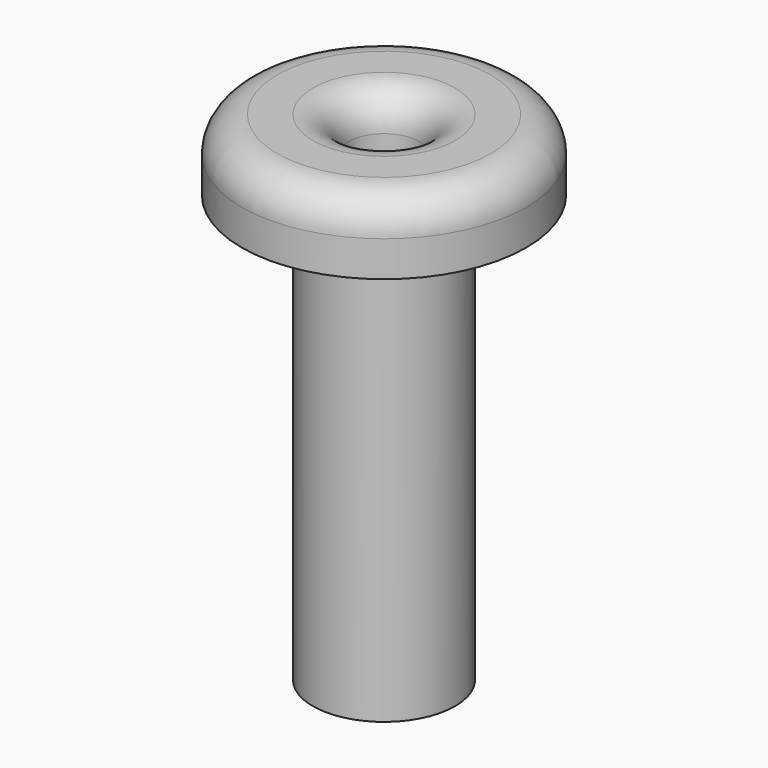
from build123d import *

# Parameters (mm, degrees)
F0_R     = 10
F0_R_2   = 2.5
F1_DEPTH = 5
F2_R     = 5
F2_R_2   = 2.5
F3_DEPTH = 30
F4_R     = 2.49999


# Not quite as in the source:
# - a fillet or chamfer is up to 0.001 mm smaller than in the source, because OpenCascade refuses the exact size


with BuildPart() as f1:
    # F0 (on Top) → F1 (new body)
    with BuildSketch(Plane.XY):
        Circle(F0_R)
        Circle(F0_R_2, mode=Mode.SUBTRACT)
    extrude(amount=F1_DEPTH)

    # F2 (on face) → F3 (join)
    with BuildSketch(Plane(origin=(0, 0, 0), x_dir=(1, 0, 0), z_dir=(0, 0, -1))):
        Circle(F2_R)
        Circle(F2_R_2, mode=Mode.SUBTRACT)
    extrude(amount=F3_DEPTH)

    # F4 (radius 2.5 in the source; OpenCascade refuses exactly that, so slightly less here)
    f4_edges = [f1.edges().sort_by_distance(p)[0] for p in [
        (-10, 0, 5),
        (-2.5, 0, 5),
        (-2.5, 0, -30),
    ]]
    fillet(f4_edges, radius=F4_R)


solid = f1.part
